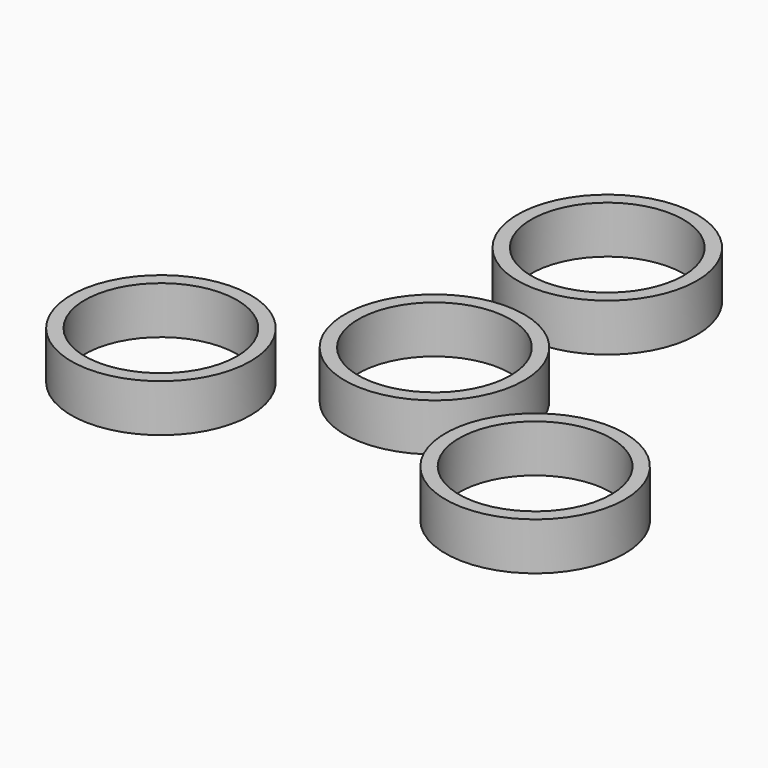
from build123d import *

# Parameters (mm, degrees)
F0_R     = 13.2
F0_R_2   = 11.2
F2_DEPTH = 7


# Not quite as in the source:
# - the program builds the solid bodies; features that only make, move or delete a surface that nothing else refers to are left out


with BuildPart() as f2:
    # F0 (on Top) → F2 (new body)
    with BuildSketch(Plane.XY):
        with Locations((0, 31.8009220064)):
            Circle(F0_R)
        with Locations((0, 31.8009220064)):
            Circle(F0_R_2, mode=Mode.SUBTRACT)
    extrude(amount=F2_DEPTH)


with BuildPart() as f2b:
    # F0 (on Top) → F2, piece 2 (new body)
    with BuildSketch(Plane.XY):
        with Locations((27.5404063213, -15.9004610032)):
            Circle(F0_R)
        with Locations((27.5404063213, -15.9004610032)):
            Circle(F0_R_2, mode=Mode.SUBTRACT)
    extrude(amount=F2_DEPTH)


with BuildPart() as f2c:
    # F0 (on Top) → F2, piece 3 (new body)
    with BuildSketch(Plane.XY):
        Circle(F0_R)
        Circle(F0_R_2, mode=Mode.SUBTRACT)
    extrude(amount=F2_DEPTH)


with BuildPart() as f2d:
    # F0 (on Top) → F2, piece 4 (new body)
    with BuildSketch(Plane.XY):
        with Locations((-27.5404063213, -15.9004610032)):
            Circle(F0_R)
        with Locations((-27.5404063213, -15.9004610032)):
            Circle(F0_R_2, mode=Mode.SUBTRACT)
    extrude(amount=F2_DEPTH)


solid = Compound([f2.part, f2b.part, f2c.part, f2d.part])
